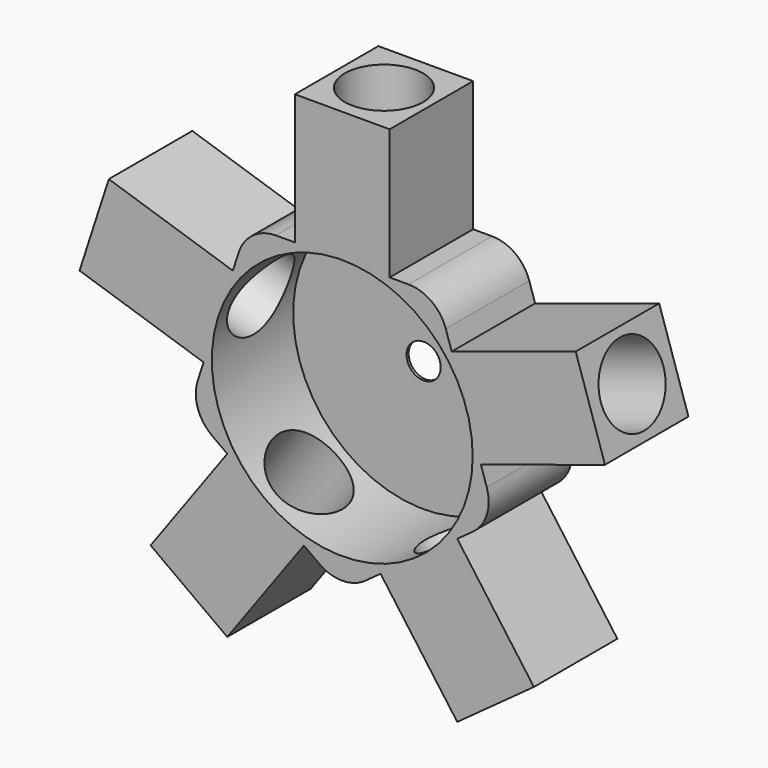
from build123d import *

# Parameters (mm, degrees)
F1_DEPTH  = 50.8
F2_R      = 63.5
F3_DEPTH  = 49.53
F4_R      = 8.3185
F5_DEPTH  = 25.4
F9_R      = 19.05
F11_DEPTH = 76.2
F10_R     = 19.05
F12_DEPTH = 76.2
F6_R      = 19.05
F13_DEPTH = 76.2
F7_R      = 19.05
F14_DEPTH = 76.2
F8_R      = 19.05
F15_DEPTH = 76.2
F16_R     = 19.05


# Not quite as in the source:
# - a feature names something its author has since deleted; it is built from what else it names


with BuildPart() as f1:
    # F0 (on Front) → F1 (new body)
    with BuildSketch(Plane.XZ):
        Polygon((-23.0722505283, 63.5), (-46.1354505283, 63.5), (-53.262371273, 41.5655933534), (-113.6544600578, 61.1881724962), (-127.9083015471, 17.319359203), (-67.5218062965, -2.3204350678), (-74.6487270411, -24.2548417144), (-55.9902062965, -37.8110505451), (-93.314569817, -89.1836296879), (-55.9828842652, -116.3066868834), (-18.6585207447, -64.9341077406), (0, -78.4903165712), (18.6585207447, -64.9341077406), (55.9828842652, -116.3066868834), (93.2999257546, -89.194269222), (55.9902062965, -37.8110505451), (74.6487270411, -24.2548417144), (67.5218062965, -2.3204350678), (127.9138950812, 17.302144075), (113.6564223157, 61.1821332873), (53.2643335309, 41.5595541445), (46.1354505283, 63.5), (23.0722505283, 63.5), (23.0722505283, 127), (-23.0722505283, 127), align=None)
    extrude(amount=F1_DEPTH)

    # F2 (on face) → F3 (cut)
    with BuildSketch(Plane.XZ.offset(50.8)):
        Circle(F2_R)
    extrude(amount=-F3_DEPTH, mode=Mode.SUBTRACT)

    # F4 (on face) → F5 (cut)
    with BuildSketch(Plane(origin=(0, 0, 0), x_dir=(-1, 0, 0), z_dir=(0, 1, 0))):
        Circle(F4_R)
    extrude(amount=-F5_DEPTH, mode=Mode.SUBTRACT)

    # F9 (on face) → F11 (cut)
    with BuildSketch(Plane(origin=(-74.6487270411, 0, -102.7451582856), x_dir=(0.8090169944, 0, -0.5877852523), z_dir=(-0.5877852523, 0, -0.8090169944))):
        with Locations((0, 25.4)):
            Circle(F9_R)
    extrude(amount=-F11_DEPTH, mode=Mode.SUBTRACT)

    # F10 (on face) → F12 (cut)
    with BuildSketch(Plane(origin=(-120.7841775695, 0, 39.2451582856), x_dir=(0, -1, 0), z_dir=(-0.9510565163, 0, 0.3090169944))):
        with Locations((25.4, 0)):
            Circle(F10_R)
    extrude(amount=-F12_DEPTH, mode=Mode.SUBTRACT)

    # F6 (on face) → F13 (cut)
    with BuildSketch(Plane.XY.offset(127)):
        with Locations((0, -25.4)):
            Circle(F6_R)
    extrude(amount=-F13_DEPTH, mode=Mode.SUBTRACT)

    # F7 (on face) → F14 (cut)
    with BuildSketch(Plane(origin=(120.7841775695, 0, 39.2451582856), x_dir=(0, 1, 0), z_dir=(0.9510565163, 0, 0.3090169944))):
        with Locations((-25.4, 0)):
            Circle(F7_R)
    extrude(amount=-F14_DEPTH, mode=Mode.SUBTRACT)

    # F8 (on face) → F15 (cut)
    with BuildSketch(Plane(origin=(74.6487270411, 0, -102.7451582856), x_dir=(0.8090169944, 0, 0.5877852523), z_dir=(0.5877852523, 0, -0.8090169944))):
        with Locations((0, 25.4)):
            Circle(F8_R)
    extrude(amount=-F15_DEPTH, mode=Mode.SUBTRACT)

    # F16
    f16_edges = [f1.edges().sort_by_distance(p)[0] for p in [
        (0, -25.4, -78.490317),
        (74.648727, -25.4, -24.254842),
        (-74.648727, -25.4, -24.254842),
        (-46.135451, -25.4, 63.5),
        (46.135451, -25.4, 63.5),
    ]]
    fillet(f16_edges, radius=F16_R)


solid = f1.part
